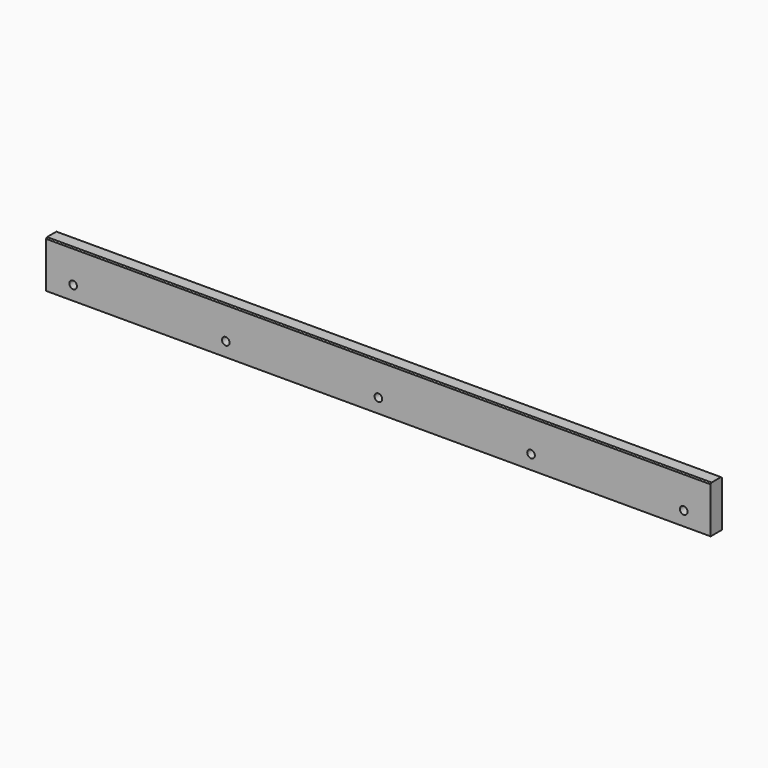
from build123d import *

# Parameters (mm, degrees)
F0_W     = 38.1
F0_H     = 127
F1_DEPTH = 898.525
F2_SIZE  = 3.175
F4_D     = 20.6375


# Not quite as in the source:
# - a length typed as a fraction of an inch, garbled in the dataset ("3 / 203.2 mm" for 3/8 in), is restored


with BuildPart() as f1:
    # F0 (on Right) → F1 (new body, symmetric)
    with BuildSketch(Plane.YZ):
        Rectangle(F0_W, F0_H)
    extrude(amount=F1_DEPTH, both=True)

    # F2
    f2_edges = [f1.edges().sort_by_distance(p)[0] for p in [
        (0, 19.05, 63.5),
        (0, -19.05, 63.5),
    ]]
    chamfer(f2_edges, length=F2_SIZE)

    # F4 (through all)
    with Locations(Plane(origin=(0, 19.05, 0), x_dir=(-1, 0, 0), z_dir=(0, 1, 0))):
        with Locations((-825.627, -25.4), (-412.877, -25.4), (-0.127, -25.4), (412.623, -25.4), (825.373, -25.4)):
            Hole(F4_D / 2)


solid = f1.part
